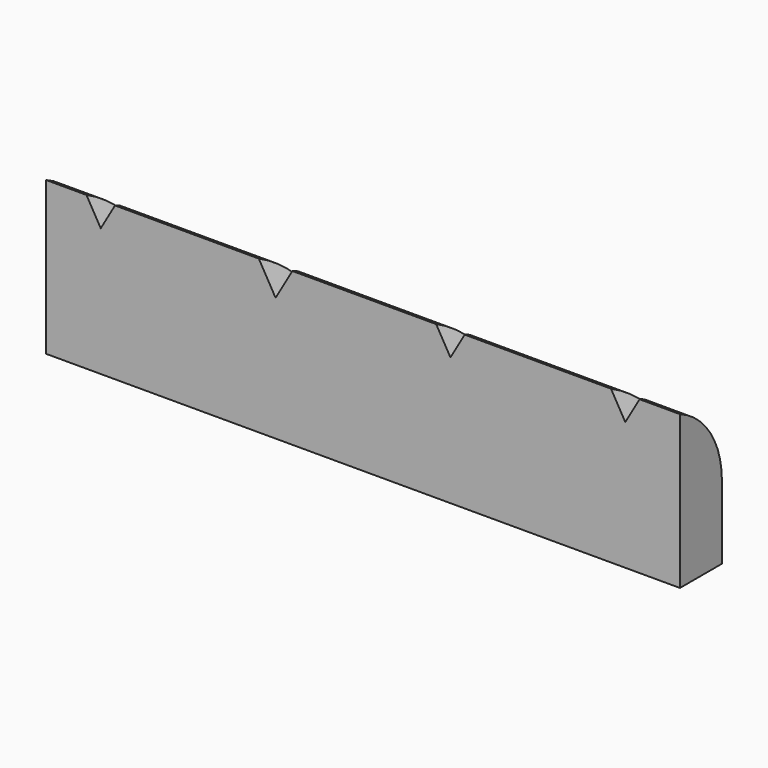
from build123d import *

# Parameters (mm, degrees)
F0_W        = 36.83
F0_H        = 3.048
F1_DEPTH    = 8.89
F3_T1_DEPTH = 60.1094845304
F4_DEPTH    = 25.4


# Not quite as in the source:
# - a fillet or chamfer that OpenCascade refuses, or shapes differently, is made with other operations: its cross-section is extruded or revolved along the edge and cut away or added


with BuildPart() as f1:
    # F0 (on Top) → F1 (new body)
    with BuildSketch(Plane.XY):
        with Locations((-0.254, 1.524)):
            Rectangle(F0_W, F0_H)
    extrude(amount=F1_DEPTH)

    # F3: fillet of radius 5.08 on 1 edges, made by hand

    # F3_s2 → F3_t1 (cut)
    with BuildSketch(Plane.YZ.offset(-30.3087422652)):
        with BuildLine():
            ThreePointArc((3.048, 4.2341030939), (2.2182329348, 7.0165336861), (0, 8.89))
            Line((0, 8.89), (3.048, 8.89))
            Line((3.048, 8.89), (3.048, 4.2341030939))
        make_face()
    extrude(amount=F3_T1_DEPTH, mode=Mode.SUBTRACT)

    # F2 (on face) → F4 (cut)
    with BuildSketch(Plane.XZ):
        Polygon((-15.494, 7.4522954744), (-14.6639409051, 8.89), (-16.3240590949, 8.89), align=None)
        Polygon((-4.3572939367, 8.89), (-6.3107060633, 8.89), (-5.334, 7.1982954744), align=None)
        Polygon((5.6560590949, 8.89), (3.9959409051, 8.89), (4.826, 7.4522954744), align=None)
        Polygon((15.8160590949, 8.89), (14.1559409051, 8.89), (14.986, 7.4522954744), align=None)
    extrude(amount=-F4_DEPTH, mode=Mode.SUBTRACT)


solid = f1.part
